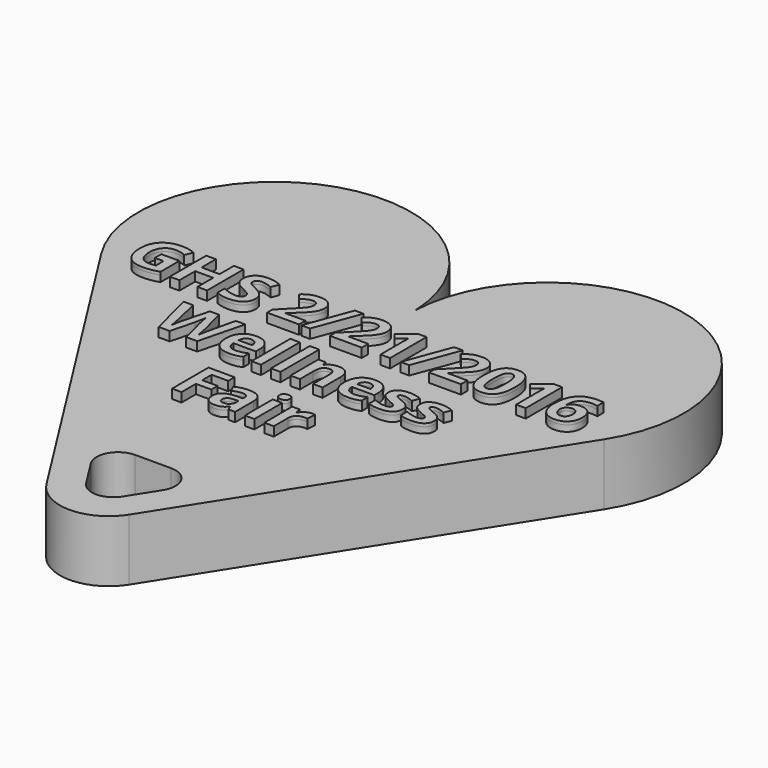
from build123d import *

# Parameters (mm, degrees)
F1_DEPTH     = 2.0134
F3_DEPTH     = 2.0134
F4_R         = 0.7
F5_TEXT_SIZE = 2.0833333333
F6_DEPTH     = 0.2
F7_R         = 1.6
F8_DEPTH     = 0.3


# Not quite as in the source:
# - Text() gives the source's letters only with a copy of the font that has no kerning and outlines rounded to 1/6400 em; it was checked with that copy


with BuildPart() as f1:
    # F0 (on Top) → F1 (new body)
    with BuildSketch(Plane.XY):
        with BuildLine():
            ThreePointArc((8.2089701458, 2.4076948693), (5.787514773, 9.0407628365), (0, 4.9953074194))
            ThreePointArc((0, 4.9953074194), (-5.787514773, 9.0407628365), (-8.2089701458, 2.4076948693))
            Line((-8.2089701458, 2.4076948693), (0, -10.5304745957))
            Line((0, -10.5304745957), (8.2089701458, 2.4076948693))
        make_face()
        with BuildLine():
            ThreePointArc((0, 4.9953074194), (0.004575039, 4.7934983507), (0, 4.5916892819))
            ThreePointArc((0, 4.5916892819), (-0.004575039, 4.7934983507), (0, 4.9953074194))
        make_face(mode=Mode.SUBTRACT)
        with BuildLine():
            ThreePointArc((0, 4.9953074194), (-0.004575039, 4.7934983507), (0, 4.5916892819))
            ThreePointArc((0, 4.5916892819), (0.004575039, 4.7934983507), (0, 4.9953074194))
        make_face()
    extrude(amount=F1_DEPTH)

    # F2 (on face) → F3 (cut, through all)
    with BuildSketch(Plane.XY.offset(2.0134)):
        Polygon((-1.8605824449, -5.7314347281), (0, -8.6639013528), (1.8605824449, -5.7314347281), align=None)
    extrude(amount=-F3_DEPTH, mode=Mode.SUBTRACT)

    # F4
    f4_edges = [f1.edges().sort_by_distance(p)[0] for p in [
        (-1.860582, -5.731435, 1.0067),
        (1.860582, -5.731435, 1.0067),
        (0, -8.663901, 1.0067),
    ]]
    fillet(f4_edges, radius=F4_R)

    # F5 (on face) → F6 (join)
    with BuildSketch(Plane.XY.offset(2.0134)):
        with Locations((-7.3852539063, 2.0560546338)):
            Text('GHS 2/21/2016', F5_TEXT_SIZE, font='Open Sans', font_style=FontStyle.BOLD, text_align=(TextAlign.LEFT, TextAlign.BOTTOM))
        with Locations((-4.5541992187, -0.2879845397)):
            Text('Wellness', F5_TEXT_SIZE, font='Open Sans', font_style=FontStyle.BOLD, text_align=(TextAlign.LEFT, TextAlign.BOTTOM))
        with Locations((-1.9700520833, -2.7354587213)):
            Text('Fair', F5_TEXT_SIZE, font='Open Sans', font_style=FontStyle.BOLD, text_align=(TextAlign.LEFT, TextAlign.BOTTOM))
    extrude(amount=F6_DEPTH)

    # F7
    f7_edges = [f1.edges().sort_by_distance(p)[0] for p in [
        (0, -10.530475, 1.0067),
    ]]
    fillet(f7_edges, radius=F7_R)

    # F5 (on face) → F8 (join)
    with BuildSketch(Plane.XY.offset(2.0134)):
        with Locations((-7.3852539063, 2.0560546338)):
            Text('GHS 2/21/2016', F5_TEXT_SIZE, font='Open Sans', font_style=FontStyle.BOLD, text_align=(TextAlign.LEFT, TextAlign.BOTTOM))
        with Locations((-4.5541992187, -0.2879845397)):
            Text('Wellness', F5_TEXT_SIZE, font='Open Sans', font_style=FontStyle.BOLD, text_align=(TextAlign.LEFT, TextAlign.BOTTOM))
        with Locations((-1.9700520833, -2.7354587213)):
            Text('Fair', F5_TEXT_SIZE, font='Open Sans', font_style=FontStyle.BOLD, text_align=(TextAlign.LEFT, TextAlign.BOTTOM))
    extrude(amount=F8_DEPTH)


solid = f1.part
